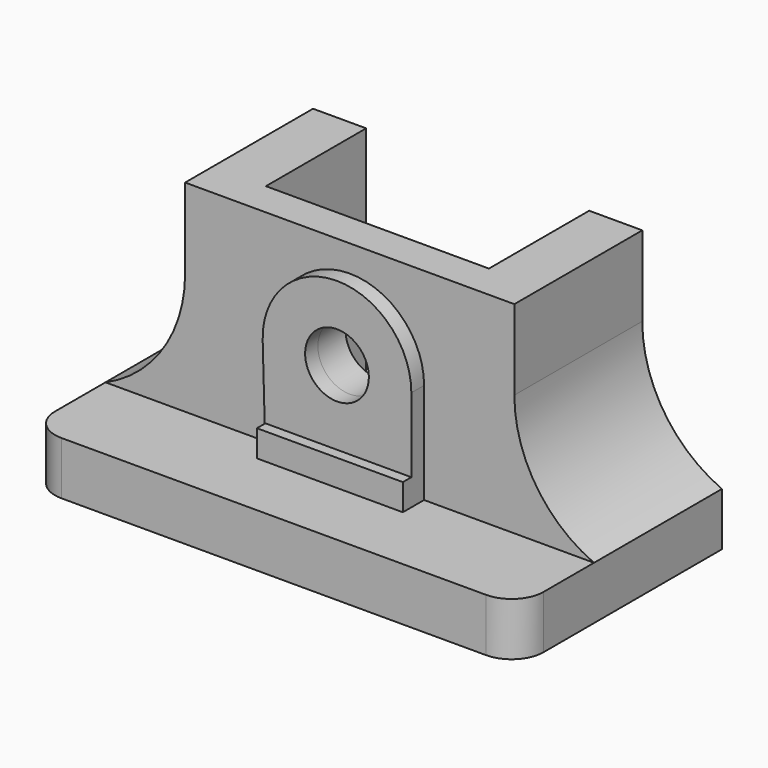
from build123d import *

# Parameters (mm, degrees)
F2_DEPTH    = 10
F3_DEPTH    = 48
F4_R        = 6
F5_DEPTH    = 3
F6_W        = 27.4810515978
F6_H        = 5
F7_DEPTH    = 2
F8_DEPTH    = 20
F9_T1_DEPTH = 30.1119658546
F10_R       = 6


# Not quite as in the source:
# - a fillet or chamfer that OpenCascade refuses, or shapes differently, is made with other operations: its cross-section is extruded or revolved along the edge and cut away or added


with BuildPart() as f2:
    # F0 (on Top) → F2 (new body)
    with BuildSketch(Plane.XY):
        Polygon((46, -18), (46, 30), (31, 30), (31, -0.1119658546), (-31, -0.1119658546), (-31, 30), (-46, 30), (-46, -18), align=None)
        Polygon((31, -0.1119658546), (31, 30), (21, 30), (21, 6.4026141707), (-21, 6.4026141707), (-21, 30), (-31, 30), (-31, -0.1119658546), align=None)
    extrude(amount=F2_DEPTH)

    # F1 (on Top) → F3 (join)
    with BuildSketch(Plane.XY):
        Polygon((31, -0.1119658546), (31, 30), (21, 30), (21, 6.4026141707), (-21, 6.4026141707), (-21, 30), (-31, 30), (-31, -0.1119658546), align=None)
    extrude(amount=F3_DEPTH)

    # F4 (on face) → F5 (join)
    with BuildSketch(Plane.XZ.offset(0.1119658546)):
        with BuildLine():
            Line((14, 10), (14, 29))
            ThreePointArc((14, 29), (-0.1930996384, 42.9986682413), (-13.9946732185, 28.6138374607))
            Line((-13.9946732185, 28.6138374607), (-13.4810515978, 10))
            Line((-13.4810515978, 10), (14, 10))
        make_face()
        with Locations((0, 29)):
            Circle(F4_R, mode=Mode.SUBTRACT)
    extrude(amount=F5_DEPTH)

    # F6 (on face) → F7 (join)
    with BuildSketch(Plane.XZ.offset(3.1119658546)):
        with Locations((0.2594742011, 12.5)):
            Rectangle(F6_W, F6_H)
    extrude(amount=F7_DEPTH)

    # F8 (cut): a face of the model
    f8_faces = [f2.faces().sort_by_distance(p)[0] for p in [
        (0, -0.1119658546, 29),
    ]]
    extrude(f8_faces, amount=-F8_DEPTH, mode=Mode.SUBTRACT)

    # F9: fillet of radius 25 on 2 edges, made by hand

    # F9_s2 → F9_t1 (join)
    with BuildSketch(Plane.XZ.offset(-30)):
        with BuildLine():
            ThreePointArc((46, 10), (35.0834993366, 19.2198145372), (31, 32.9128784748))
            Line((31, 32.9128784748), (31, 10))
            Line((31, 10), (46, 10))
        make_face()
        with BuildLine():
            ThreePointArc((-46, 10), (-35.0834993366, 19.2198145372), (-31, 32.9128784748))
            Line((-31, 32.9128784748), (-31, 10))
            Line((-31, 10), (-46, 10))
        make_face()
    extrude(amount=F9_T1_DEPTH)

    # F10
    f10_edges = [f2.edges().sort_by_distance(p)[0] for p in [
        (-46, -18, 5),
        (46, -18, 5),
    ]]
    fillet(f10_edges, radius=F10_R)


solid = f2.part
